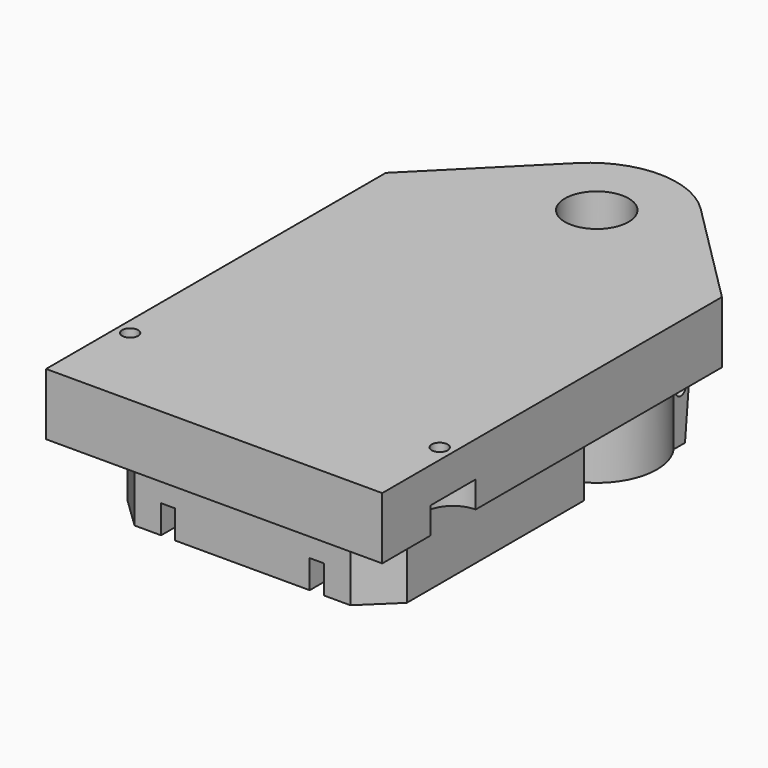
from build123d import *

# Parameters (mm, degrees)
F0_R      = 4.5
F1_DEPTH  = 35
F2_DEPTH  = 24
F3_DEPTH  = 15
F5_DEPTH  = 35
F7_DEPTH  = 83
F9_DEPTH  = 290
F10_R     = 18
F11_DEPTH = 199
F12_W     = 2.5
F12_H     = 32
F13_DEPTH = 40
F8_R      = 3.5
F14_DEPTH = 99.1
F15_W     = 76
F15_H     = 160
F16_DEPTH = 16
F17_DEPTH = 24


# Not quite as in the source:
# - a feature names something its author has since deleted; it is built from what else it names


with BuildPart() as f1:
    # F0 (on Top) → F1 (new body)
    with BuildSketch(Plane.XY):
        with BuildLine():
            Line((95, 100), (35, 160))
            Line((35, 160), (-35, 160))
            Line((-35, 160), (-95, 100))
            Line((-95, 100), (-95, -74))
            ThreePointArc((-95, -74), (-83.686291501, -78.686291501), (-79, -90))
            Line((-79, -90), (-79, 40))
            Line((-79, 40), (79, 40))
            Line((79, 40), (79, -90))
            ThreePointArc((79, -90), (83.686291501, -78.686291501), (95, -74))
            Line((95, -74), (95, 100))
        make_face()
        with BuildLine():
            Line((95, -140), (95, -106))
            ThreePointArc((95, -106), (83.686291501, -101.313708499), (79, -90))
            Line((79, -90), (79, -120))
            Line((79, -120), (-79, -120))
            Line((-79, -120), (-79, -90))
            ThreePointArc((-79, -90), (-83.686291501, -101.313708499), (-95, -106))
            Line((-95, -106), (-95, -140))
            Line((-95, -140), (95, -140))
        make_face()
        with BuildLine():
            ThreePointArc((-79, -90), (-83.686291501, -78.686291501), (-95, -74))
            Line((-95, -74), (-95, -106))
            ThreePointArc((-95, -106), (-83.686291501, -101.313708499), (-79, -90))
        make_face()
        with Locations((-87.5, -90)):
            Circle(F0_R, mode=Mode.SUBTRACT)
        with BuildLine():
            Line((95, -106), (95, -74))
            ThreePointArc((95, -74), (83.686291501, -78.686291501), (79, -90))
            ThreePointArc((79, -90), (83.686291501, -101.313708499), (95, -106))
        make_face()
        with Locations((87.5, -90)):
            Circle(F0_R, mode=Mode.SUBTRACT)
        Polygon((79, -120), (79, -90), (79, 40), (-79, 40), (-79, -90), (-79, -120), align=None)
    extrude(amount=F1_DEPTH)

    # F0 (on Top) → F2 (join)
    with BuildSketch(Plane.XY):
        Polygon((79, -120), (79, -90), (79, 40), (-79, 40), (-79, -90), (-79, -120), align=None)
    extrude(amount=-F2_DEPTH)

    # F0 (on Top) → F3 (cut)
    with BuildSketch(Plane.XY):
        with BuildLine():
            ThreePointArc((-79, -90), (-83.686291501, -78.686291501), (-95, -74))
            Line((-95, -74), (-95, -106))
            ThreePointArc((-95, -106), (-83.686291501, -101.313708499), (-79, -90))
        make_face()
        with Locations((-87.5, -90)):
            Circle(F0_R, mode=Mode.SUBTRACT)
        with BuildLine():
            Line((95, -106), (95, -74))
            ThreePointArc((95, -74), (83.686291501, -78.686291501), (79, -90))
            ThreePointArc((79, -90), (83.686291501, -101.313708499), (95, -106))
        make_face()
        with Locations((87.5, -90)):
            Circle(F0_R, mode=Mode.SUBTRACT)
    extrude(amount=F3_DEPTH, mode=Mode.SUBTRACT)

    # F4 (on face) → F5 (join)
    with BuildSketch(Plane(origin=(0, 0, 0), x_dir=(1, 0, 0), z_dir=(0, 0, -1))):
        with BuildLine():
            Line((35, -160), (-35, -160))
            ThreePointArc((-35, -160), (0, -174.4974746831), (35, -160))
        make_face()
    extrude(amount=-F5_DEPTH)

    # F6 (on face) → F7 (join)
    with BuildSketch(Plane(origin=(0, 0, 0), x_dir=(1, 0, 0), z_dir=(0, 0, -1))):
        with BuildLine():
            Line((-27.7308492477, -166), (27.7308492477, -166))
            Line((27.7308492477, -166), (27.7308492477, -150))
            ThreePointArc((27.7308492477, -150), (0, -96.3276844271), (-27.7308492477, -150))
            Line((-27.7308492477, -150), (-27.7308492477, -166))
        make_face()
    extrude(amount=F7_DEPTH)

    # F8 (on face) → F9 (cut)
    with BuildSketch(Plane(origin=(-27.7308492477, 0, 0), x_dir=(0, -1, 0), z_dir=(-1, 0, 0))):
        Polygon((-158, -83), (-166, 0), (-166, -83), align=None)
    extrude(amount=-F9_DEPTH, mode=Mode.SUBTRACT)

    # F10 (on face) → F11 (cut)
    with BuildSketch(Plane(origin=(0, 0, -83), x_dir=(1, 0, 0), z_dir=(0, 0, -1))):
        with Locations((0, -130.3276844271)):
            Circle(F10_R)
    extrude(amount=-F11_DEPTH, mode=Mode.SUBTRACT)

    # F12 (on face) → F13 (cut)
    with BuildSketch(Plane(origin=(0, 0, -83), x_dir=(1, 0, 0), z_dir=(0, 0, -1))):
        with Locations((0, -174)):
            Rectangle(F12_W, F12_H)
        with BuildLine():
            ThreePointArc((1.25, -148.2842291949), (0, -148.3276844271), (-1.25, -148.2842291949))
            Line((-1.25, -148.2842291949), (-1.25, -158))
            Line((-1.25, -158), (1.25, -158))
            Line((1.25, -158), (1.25, -148.2842291949))
        make_face()
    extrude(amount=-F13_DEPTH, mode=Mode.SUBTRACT)

    # F8 (on face) → F14 (cut)
    with BuildSketch(Plane(origin=(-27.7308492477, 0, 0), x_dir=(0, -1, 0), z_dir=(-1, 0, 0))):
        with Locations((-155, -55)):
            Circle(F8_R)
    extrude(amount=-F14_DEPTH, mode=Mode.SUBTRACT)

    # F15 (on face) → F16 (join)
    with BuildSketch(Plane(origin=(0, 0, -24), x_dir=(1, 0, 0), z_dir=(0, 0, -1))):
        Polygon((-46, -40), (-46, 120), (-61, 120), (-79, 102.6506484271), (-79, -22.6506484271), (-61, -40), align=None)
        with Locations((0, 40)):
            Rectangle(F15_W, F15_H)
        Polygon((61, 120), (46, 120), (46, -40), (61, -40), (79, -22.6506484271), (79, 102.6506484271), align=None)
    extrude(amount=F16_DEPTH)

    # F15 (on face) → F17 (cut)
    with BuildSketch(Plane(origin=(0, 0, -24), x_dir=(1, 0, 0), z_dir=(0, 0, -1))):
        Polygon((-79, -40), (-61, -40), (-79, -22.6506484271), align=None)
        Polygon((-79, 102.6506484271), (-61, 120), (-79, 120), align=None)
        Polygon((79, 120), (61, 120), (79, 102.6506484271), align=None)
        Polygon((79, -22.6506484271), (61, -40), (79, -40), align=None)
    extrude(amount=-F17_DEPTH, mode=Mode.SUBTRACT)


solid = f1.part
